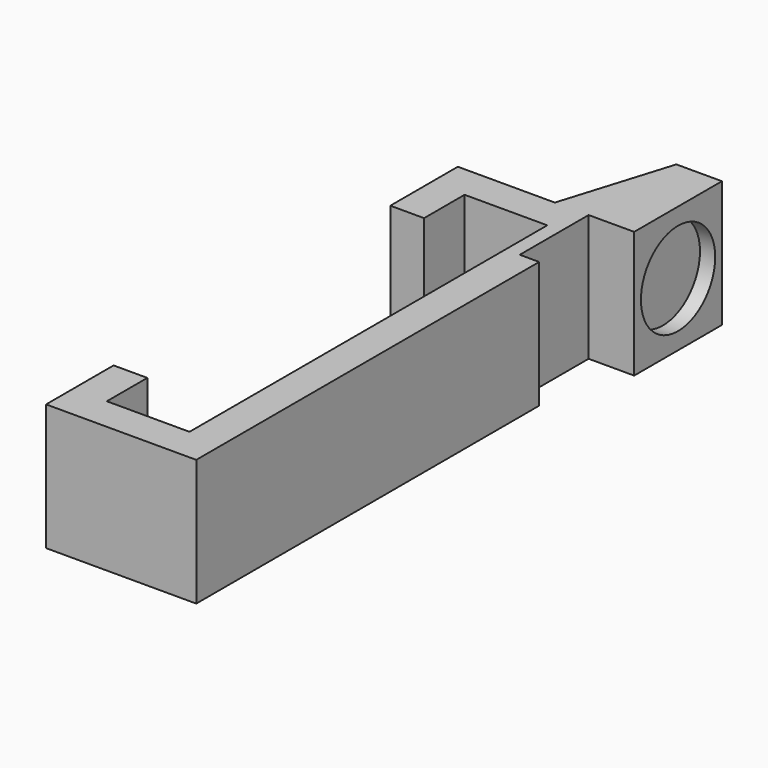
from build123d import *

# Parameters (mm, degrees)
F0_W     = 2.3
F0_H     = 4
F0_W_2   = 5.4
F0_H_2   = 13
F0_W_3   = 1.7
F0_H_3   = 46.8
F0_W_4   = 4
F0_H_4   = 6
F1_DEPTH = 15
F2_R     = 5.5
F3_DEPTH = 1.8


# Not quite as in the source:
# - a feature names something its author has since deleted; it is built from what else it names


with BuildPart() as f1:
    # F0 (on Top) → F1 (new body)
    with BuildSketch(Plane.XY):
        Polygon((0, -23.2), (0, -13), (-1.7, -13), (-1.7, -17), (-1.7, -23.2), align=None)
        with Locations((-2.85, -15)):
            Rectangle(F0_W, F0_H)
        with Locations((2.7, -6.5)):
            Rectangle(F0_W_2, F0_H_2)
        with Locations((-0.85, -46.6)):
            Rectangle(F0_W_3, F0_H_3)
        Polygon((-11.5, -74), (-11.5, -70), (-11.5, -64), (-15.5, -64), (-15.5, -74), align=None)
        with Locations((1.15, -46.6)):
            Rectangle(F0_W, F0_H_3)
        Polygon((2.3, -70), (0, -70), (-1.7, -70), (-11.5, -70), (-11.5, -74), (2.3, -74), align=None)
        Polygon((0, -13), (0, 0), (-4, -13), (-1.7, -13), align=None)
        Polygon((-4, -17), (-4, -13), (-15.5, -13), (-15.5, -17), (-11.5, -17), align=None)
        with Locations((-13.5, -20)):
            Rectangle(F0_W_4, F0_H_4)
    extrude(amount=F1_DEPTH)

    # F2 (on face) → F3 (cut)
    with BuildSketch(Plane.YZ.offset(5.4)):
        with Locations((-6.5, 7.5)):
            Circle(F2_R)
    extrude(amount=-F3_DEPTH, mode=Mode.SUBTRACT)


solid = f1.part
